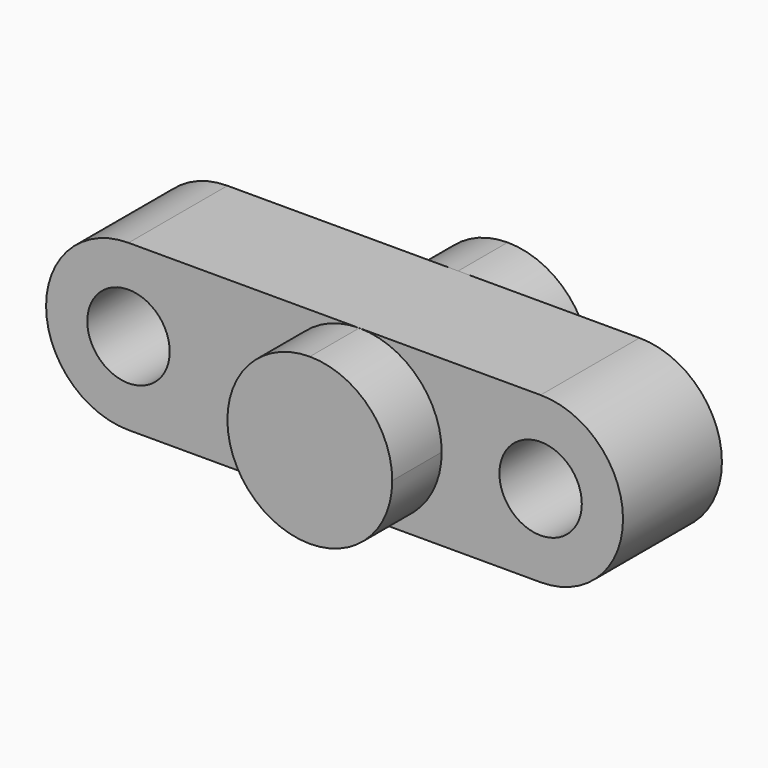
from build123d import *

# Parameters (mm, degrees)
F0_R          = 0.5
F1_DEPTH      = 1.5
F2_DEPTH      = 0.75
F2_DEPTH_BACK = 2.25


# Not quite as in the source:
# - a feature names something its author has since deleted; it is built from what else it names


with BuildPart() as f1:
    # F0 (on Front) → F1 (new body)
    with BuildSketch(Plane.XZ):
        with BuildLine():
            ThreePointArc((-2.2, -2.1902196236), (-3.2, -1.1902196236), (-2.2, -0.1902196236))
            Line((-2.2, -0.1902196236), (-2.8, -0.1902196236))
            ThreePointArc((-2.8, -0.1902196236), (-3.8, -1.1902196236), (-2.8, -2.1902196236))
            Line((-2.8, -2.1902196236), (-2.2, -2.1902196236))
        make_face()
        with BuildLine():
            Line((0, -0.1902196236), (-2.2, -0.1902196236))
            ThreePointArc((-2.2, -0.1902196236), (-1.4928932188, -0.4831128424), (-1.2, -1.1902196236))
            ThreePointArc((-1.2, -1.1902196236), (-1.4928932188, -1.8973264048), (-2.2, -2.1902196236))
            Line((-2.2, -2.1902196236), (0, -2.1902196236))
            ThreePointArc((0, -2.1902196236), (1, -1.1902196236), (0, -0.1902196236))
        make_face()
        with Locations((0, -1.1902196236)):
            Circle(F0_R, mode=Mode.SUBTRACT)
        with BuildLine():
            ThreePointArc((-2.8, -2.1902196236), (-3.8, -1.1902196236), (-2.8, -0.1902196236))
            Line((-2.8, -0.1902196236), (-5, -0.1902196236))
            ThreePointArc((-5, -0.1902196236), (-6, -1.1902196236), (-5, -2.1902196236))
            Line((-5, -2.1902196236), (-2.8, -2.1902196236))
        make_face()
        with Locations((-5, -1.1902196236)):
            Circle(F0_R, mode=Mode.SUBTRACT)
        with BuildLine():
            ThreePointArc((-1.2, -1.1902196236), (-1.4928932188, -0.4831128424), (-2.2, -0.1902196236))
            ThreePointArc((-2.2, -0.1902196236), (-3.2, -1.1902196236), (-2.2, -2.1902196236))
            ThreePointArc((-2.2, -2.1902196236), (-1.4928932188, -1.8973264048), (-1.2, -1.1902196236))
        make_face()
    extrude(amount=F1_DEPTH)

    # F0 (on Front) → F2 (join, two sides)
    with BuildSketch(Plane.XZ) as f2_sk:
        with BuildLine():
            ThreePointArc((-1.2, -1.1902196236), (-1.4928932188, -0.4831128424), (-2.2, -0.1902196236))
            ThreePointArc((-2.2, -0.1902196236), (-3.2, -1.1902196236), (-2.2, -2.1902196236))
            ThreePointArc((-2.2, -2.1902196236), (-1.4928932188, -1.8973264048), (-1.2, -1.1902196236))
        make_face()
    extrude(amount=-F2_DEPTH)
    extrude(f2_sk.sketch, amount=F2_DEPTH_BACK)


solid = f1.part
